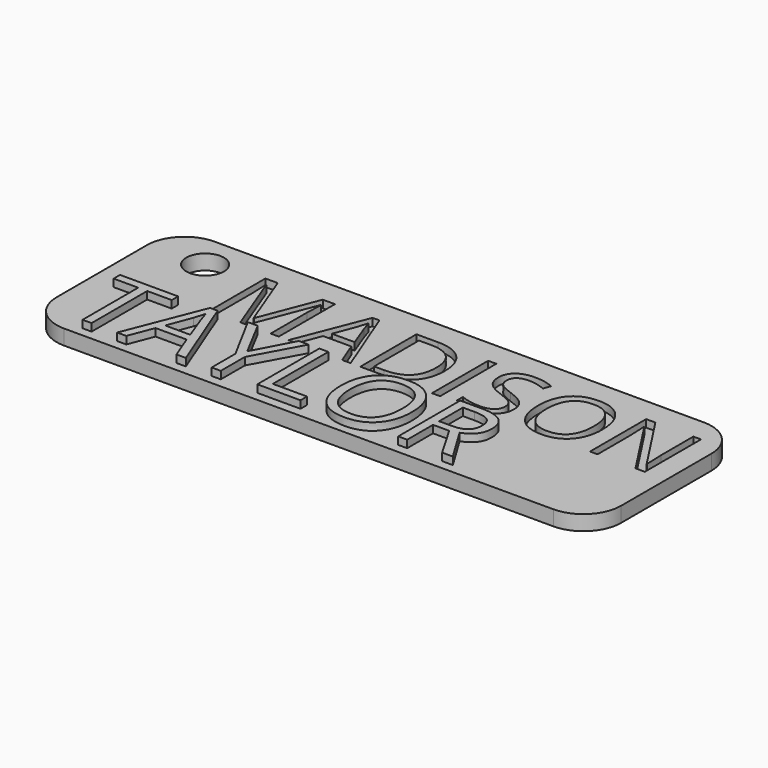
from build123d import *

# Parameters (mm, degrees)
F1_DEPTH     = 2
F3_D         = 5
F5_TEXT_SIZE = 14.4235559371
F6_DEPTH     = 1
F4_TEXT_SIZE = 13.067002416
F7_DEPTH     = 1


# Not quite as in the source:
# - Text() gives the source's letters only with a copy of the font that has no kerning and outlines rounded to 1/6400 em; it was checked with that copy


with BuildPart() as f1:
    # F0 (on Top) → F1 (new body)
    with BuildSketch(Plane.XY):
        with BuildLine():
            ThreePointArc((37.5, 7.5), (36.0355339059, 11.0355339059), (32.5, 12.5))
            Line((32.5, 12.5), (-32.5, 12.5))
            ThreePointArc((-32.5, 12.5), (-36.0355339059, 11.0355339059), (-37.5, 7.5))
            Line((-37.5, 7.5), (-37.5, -7.5))
            ThreePointArc((-37.5, -7.5), (-36.0355339059, -11.0355339059), (-32.5, -12.5))
            Line((-32.5, -12.5), (32.5, -12.5))
            ThreePointArc((32.5, -12.5), (36.0355339059, -11.0355339059), (37.5, -7.5))
            Line((37.5, -7.5), (37.5, 7.5))
        make_face()
    extrude(amount=F1_DEPTH)

    # F3 (through all)
    with Locations(Plane(origin=(0, 0, 0), x_dir=(1, 0, 0), z_dir=(0, 0, -1))):
        with Locations((-30.0543494523, -7.8623192385)):
            Hole(F3_D / 2)

    # F5 (on face) → F6 (join)
    with BuildSketch(Plane.XY.offset(2)):
        with Locations((-34.420542419, -11.2652787939)):
            Text('TAYLOR', F5_TEXT_SIZE, font='Open Sans', text_align=(TextAlign.LEFT, TextAlign.BOTTOM))
    extrude(amount=F6_DEPTH)

    # F4 (on face) → F7 (cut)
    with BuildSketch(Plane.XY.offset(2)):
        with Locations((-24.5, 0)):
            Text('MADISON', F4_TEXT_SIZE, font='Open Sans', text_align=(TextAlign.LEFT, TextAlign.BOTTOM))
    extrude(amount=-F7_DEPTH, mode=Mode.SUBTRACT)


solid = f1.part
